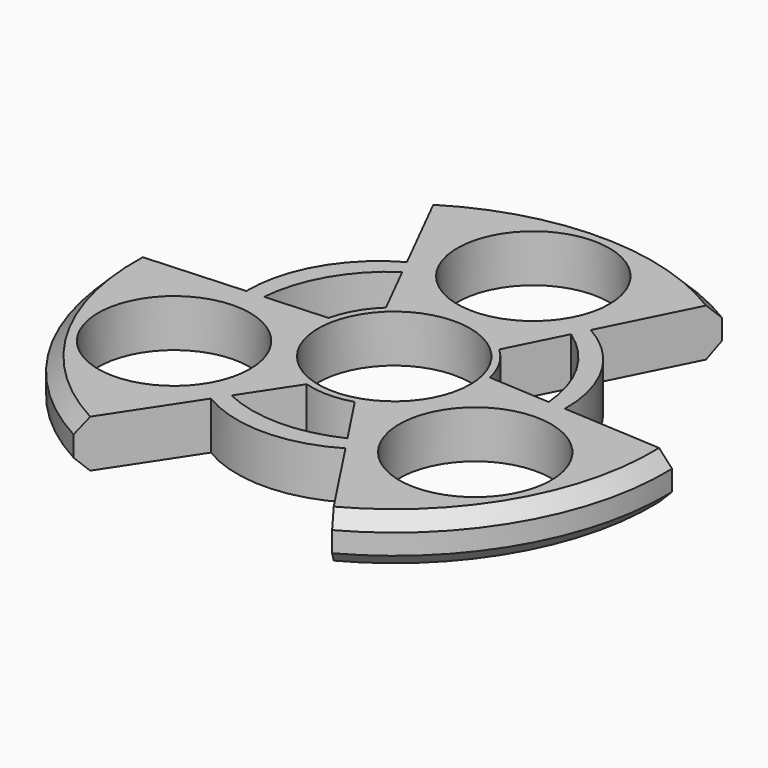
from build123d import *

# Parameters (mm, degrees)
F0_R            = 11.175
F1_DEPTH        = 7
F2_COUNT        = 3
F4_DEPTH        = 7
F4_COPIES_COUNT = 3
F5_SIZE         = 2
F6_SIZE         = 2
F7_SIZE         = 2


# Not quite as in the source:
# - a pattern or mirror of a feature is missing from the dataset's text; its kind, count and spacing are read off the source's solid


with BuildPart() as f1:
    # F0 (on Top) → F1 (new body)
    with BuildSketch(Plane.XY):
        with BuildLine():
            ThreePointArc((-8.3372222223, 8.8987877603), (-4.8493412747, -11.1884577663), (12.1941665556, 0))
            ThreePointArc((12.1941665556, 0), (11.1884577663, 4.8493412747), (8.3372222223, 8.8987877603))
            ThreePointArc((8.3372222223, 8.8987877603), (0, 12.1941665556), (-8.3372222223, 8.8987877603))
        make_face()
        Circle(F0_R, mode=Mode.SUBTRACT)
        with BuildLine():
            ThreePointArc((-8.3372222223, 8.8987877603), (0, 12.1941665556), (8.3372222223, 8.8987877603))
            Line((8.3372222223, 8.8987877603), (20.9652856439, 34.0654780954))
            ThreePointArc((20.9652856439, 34.0654780954), (0, 40.0055861953), (-20.9652856439, 34.0654780954))
            Line((-20.9652856439, 34.0654780954), (-8.3372222223, 8.8987877603))
        make_face()
        with Locations((0, 25.5817994475)):
            Circle(F0_R, mode=Mode.SUBTRACT)
    extrude(amount=F1_DEPTH)

    # F2: F1 ×3 about axis
    f2_axis = Axis((0, 0, 0), (0, 0, -1))


with BuildPart() as f1_1:
    add(f1.part)
    for i in range(1, F2_COUNT):
        add(f1.part.rotate(f2_axis, i * 360 / F2_COUNT))

    # F3 (on face) → F4 (join)
    with BuildSketch(Plane.XY.offset(7)):
        with BuildLine():
            Line((-8.5294263987, -19.2529557346), (-9.9039361375, -21.3411901509))
            ThreePointArc((-9.9039361375, -21.3411901509), (0, -24.0747086913), (9.9039361375, -21.3411901509))
            Line((9.9039361375, -21.3411901509), (8.5294263987, -19.2529557346))
            ThreePointArc((8.5294263987, -19.2529557346), (0, -21.1847607817), (-8.5294263987, -19.2529557346))
        make_face()
    f4 = extrude(amount=-F4_DEPTH)

    # F4_copies: F4 ×3 about axis
    f4_copies_axis = Axis((0, 0, 0), (0, 0, 1))
    for i in range(1, F4_COPIES_COUNT):
        add(f4.rotate(f4_copies_axis, i * 360 / F4_COPIES_COUNT))

    # F5
    f5_edges = [f1_1.edges().sort_by_distance(p)[0] for p in [
        (34.645854, -20.002793, 7),
        (34.645854, -20.002793, 0),
    ]]
    chamfer(f5_edges, length=F5_SIZE)

    # F6
    f6_edges = [f1_1.edges().sort_by_distance(p)[0] for p in [
        (-34.645854, -20.002793, 7),
        (-34.645854, -20.002793, 0),
    ]]
    chamfer(f6_edges, length=F6_SIZE)

    # F7
    f7_edges = [f1_1.edges().sort_by_distance(p)[0] for p in [
        (0, 40.005586, 7),
        (0, 40.005586, 0),
    ]]
    chamfer(f7_edges, length=F7_SIZE)


solid = f1_1.part
